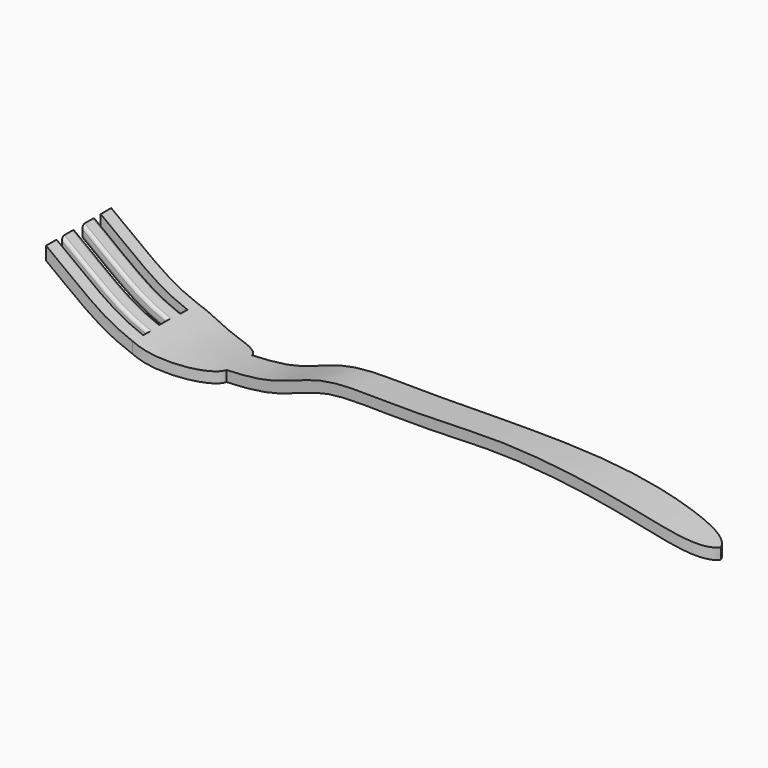
from build123d import *

# Parameters (mm, degrees)
F1_DEPTH = 25.4
F3_DEPTH = 25.908
F4_R     = 0.762


# Not quite as in the source:
# - the dataset's text gives a spline's control points without its knots; the knots are read off the source's solid


with BuildPart() as f1:
    # F0 (on Front) → F1 (new body)
    with BuildSketch(Plane.XZ):
        with BuildLine():
            add(Edge.make_bspline(
                [(0, 0), (4.7103622723, -3.4647853542), (12.9147198553, -10.1575411812), (20.8226061313, -13.5717877714), (29.1992543497, -16.2988547082), (40.8233166057, -16.1709285744), (50.5721843035, -15.0477736555), (61.1540658725, -10.0294244628), (74.311024502, -10.2781045495), (88.2869528256, -10.3453982828), (102.9561897414, -9.7815230792), (119.6924030825, -10.4922157871), (135.3180821622, -12.6217410991), (149.9409980088, -16.5686489653), (162.1173458686, -19.637861797), (165.1, -21.6453093381)],
                knots=[0, 0, 0, 0, 0.0868559245, 0.1486348932, 0.2109297072, 0.2831793526, 0.3500872914, 0.421714626, 0.4985865883, 0.5782941352, 0.6601147558, 0.7473436335, 0.8315638983, 0.9168249177, 1, 1, 1, 1], degree=3))
            Line((0, 0), (-1.5050336483, -2.0460874169))
            add(Edge.make_bspline(
                [(-1.5050336483, -2.0460874169), (0.1637206937, -3.2735674428), (3.5533400926, -5.8652853154), (7.6813245522, -9.0003571227), (10.4129282883, -10.9156588472), (11.9229553181, -11.9018082786), (13.3915322874, -12.8007225517), (15.1374988164, -13.758712094), (17.1384561844, -14.7045275776), (18.7586406624, -15.371557203), (20.0430367648, -15.8628596575), (21.3455956551, -16.3437983832), (23.0527587629, -16.9283625946), (25.237785357, -17.5589293042), (27.1890359841, -17.9919031982), (28.8403738254, -18.2630534425), (30.5400869227, -18.475599715), (32.7149442827, -18.6393564524), (35.3651435578, -18.705485202), (38.0007231957, -18.668412959), (40.1381152796, -18.5726076041), (41.7851365475, -18.4701459897), (43.4117405729, -18.3457892195), (45.4122753416, -18.1372349694), (47.7938153543, -17.7647931119), (49.5851269052, -17.3656809964), (50.7874550731, -17.0393038831), (51.5931972947, -16.8042840122), (52.9854688837, -16.3575049067), (54.9333065508, -15.6538415885), (56.8468256288, -14.9448741212), (58.3647728478, -14.4191213897), (59.497552549, -14.0559637458), (60.6274625059, -13.7334991856), (61.7490901661, -13.4624552167), (62.8881515601, -13.2460285779), (64.4563385096, -13.0181885844), (66.4922293506, -12.8389641651), (69.0431120474, -12.7526468301), (71.242678231, -12.7518730229), (73.0369209896, -12.7704698964), (74.8547509529, -12.793365858), (77.138297349, -12.8165189546), (79.8874154417, -12.8336539859), (82.6465251687, -12.8367354073), (85.4132365312, -12.8227538429), (88.1889904301, -12.7885674657), (90.9634534916, -12.7311143345), (93.7379371108, -12.6634846961), (96.5263627749, -12.598491337), (99.3400340277, -12.5488993737), (102.1896850554, -12.5269325718), (105.0923644315, -12.5461752999), (109.0305615295, -12.630891922), (114.0226244428, -12.8474654753), (119.9666981593, -13.2882856574), (124.7569495699, -13.8095922492), (128.5099304625, -14.3309214218), (131.2880701954, -14.7769525103), (134.0333704954, -15.2805454236), (136.7501374746, -15.8460323202), (139.4762553032, -16.4714574202), (142.2383592807, -17.1491776073), (145.0646471313, -17.872573562), (147.4961661466, -18.5072330209), (149.499890848, -19.0304339595), (151.5490856864, -19.5619912612), (154.1344418244, -20.2362902831), (157.1317410624, -21.0772186864), (159.8666787498, -21.9574045978), (162.1676040395, -22.8717505548), (163.2756026045, -23.479125985), (163.6817765955, -23.7524976009)],
                knots=[0, 0, 0, 0, 0.03125, 0.0625, 0.078125, 0.0859375, 0.09375, 0.109375, 0.125, 0.140625, 0.1484375, 0.15625, 0.171875, 0.1875, 0.203125, 0.2109375, 0.21875, 0.234375, 0.25, 0.265625, 0.28125, 0.2890625, 0.296875, 0.3125, 0.328125, 0.34375, 0.34765625, 0.3515625, 0.359375, 0.375, 0.390625, 0.3984375, 0.40625, 0.4140625, 0.421875, 0.4296875, 0.4375, 0.453125, 0.46875, 0.484375, 0.4921875, 0.5, 0.515625, 0.53125, 0.546875, 0.5625, 0.578125, 0.59375, 0.609375, 0.625, 0.640625, 0.65625, 0.671875, 0.6875, 0.71875, 0.75, 0.78125, 0.796875, 0.8125, 0.828125, 0.84375, 0.859375, 0.875, 0.890625, 0.90625, 0.9140625, 0.921875, 0.9375, 0.953125, 0.96875, 0.984375, 1, 1, 1, 1], degree=3))
            Line((163.6817765955, -23.7524976009), (165.1, -21.6453093381))
        make_face()
    extrude(amount=F1_DEPTH)

    # F2 (on Top) → F3 (cut)
    with BuildSketch(Plane.XY):
        Polygon((184.9420815706, 20.2900245786), (-14.0935713425, 17.0680619776), (-14.0935713425, -45.046299696), (184.9420815706, -45.046299696), align=None)
        with BuildLine():
            Line((20.5693654716, -13.7910833582), (20.5693654716, -12.7))
            Line((20.5693654716, -12.7), (20.5693654716, -11.6089166418))
            Line((20.5693654716, -11.6089166418), (0, -11.6089166418))
            Line((0, -11.6089166418), (0, -7.6876155376))
            Line((0, -7.6876155376), (20.7349956036, -7.6876155376))
            Line((20.7349956036, -7.6876155376), (20.7349956036, -6.094103986))
            Line((20.7349956036, -6.094103986), (0, -6.094103986))
            Line((0, -6.094103986), (0, -2.9581359863))
            Line((0, -2.9581359863), (20.7349956036, -2.9581359863))
            add(Edge.make_bspline(
                [(20.7349956036, -2.9581359863), (23.7156929802, -2.7633162878), (28.3999497355, -4.1187867179), (37.8254950423, -6.5219569101), (38.4486503899, -8.8805224091)],
                knots=[0, 0, 0, 0, 0.4791596741, 1, 1, 1, 1], degree=3))
            add(Edge.make_bspline(
                [(38.4486503899, -8.8805224091), (51.7361002743, -8.8956270078), (65.1850104393, -8.9186783015), (92.1523955049, -8.7511104116), (106.8150461235, -9.3737340764), (146.9355739457, -6.6714390526), (152.9013983717, -10.881973577), (153.6982059479, -12.7)],
                knots=[0, 0, 0, 0, 0.2088243882, 0.397348135, 0.5578330827, 0.8000414169, 0.9059927895, 0.9059927895, 0.9059927895, 0.9059927895], degree=3))
            add(Edge.make_bspline(
                [(38.4486503899, -16.5194775909), (51.7361002743, -16.5043729922), (65.1850104393, -16.4813216985), (92.1523955049, -16.6488895884), (106.8150461235, -16.0262659236), (146.9355739457, -18.7285609474), (152.9013983717, -14.518026423), (153.6982059479, -12.7)],
                knots=[0, 0, 0, 0, 0.2088243882, 0.397348135, 0.5578330827, 0.8000414169, 0.9059927895, 0.9059927895, 0.9059927895, 0.9059927895], degree=3))
            add(Edge.make_bspline(
                [(20.7349956036, -22.4418640137), (23.7156929802, -22.6366837122), (28.3999497355, -21.2812132821), (37.8254950423, -18.8780430899), (38.4486503899, -16.5194775909)],
                knots=[0, 0, 0, 0, 0.4791596741, 1, 1, 1, 1], degree=3))
            Line((20.7349956036, -22.4418640137), (0, -22.4418640137))
            Line((0, -22.4418640137), (0, -19.305896014))
            Line((0, -19.305896014), (20.7349956036, -19.305896014))
            Line((20.7349956036, -19.305896014), (20.7349956036, -17.7123844624))
            Line((20.7349956036, -17.7123844624), (0, -17.7123844624))
            Line((0, -17.7123844624), (0, -13.7910833582))
            Line((0, -13.7910833582), (20.5693654716, -13.7910833582))
        make_face(mode=Mode.SUBTRACT)
    extrude(amount=-F3_DEPTH, mode=Mode.SUBTRACT)

    # F4
    f4_edges = [f1.edges().sort_by_distance(p)[0] for p in [
        (9.913112, -17.712384, -7.446879),
        (9.841289, -13.791083, -7.395002),
        (9.774251, -13.791083, -10.462191),
        (9.774251, -11.608917, -10.462191),
        (9.846699, -17.712384, -10.512501),
        (9.846699, -7.687616, -10.512501),
        (9.841289, -11.608917, -7.395002),
        (9.913112, -7.687616, -7.446879),
    ]]
    fillet(f4_edges, radius=F4_R)


solid = f1.part
